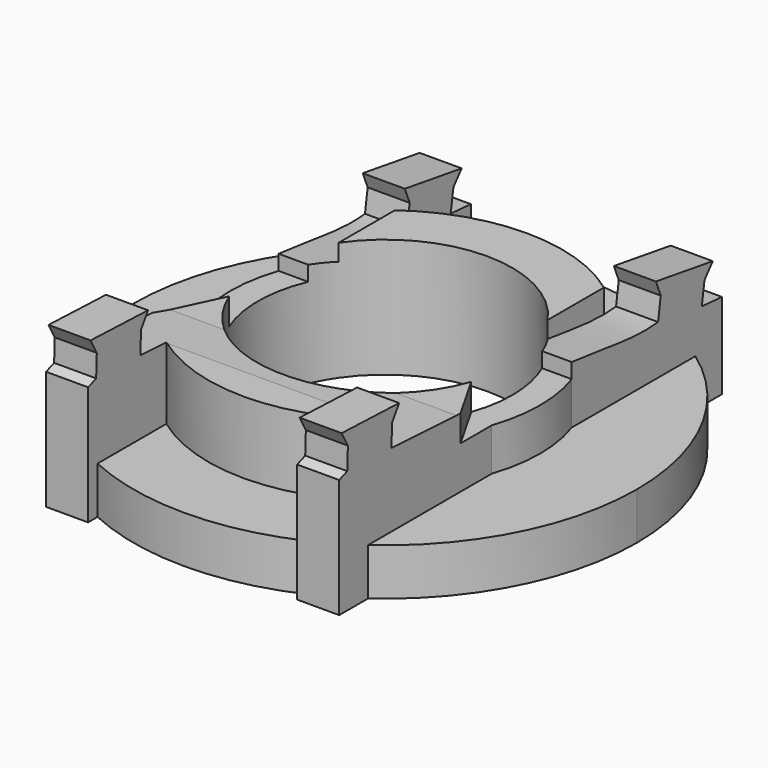
from build123d import *
from build123d import SkipClean  # not in build123d's __all__

# Parameters (mm, degrees)
F2_DEPTH = 8.5
F3_DEPTH = 29
F4_DEPTH = 16.2
F5_DEPTH = 21.5
F6_W     = 8.4938306999
F6_H     = 8
F7_DEPTH = 53
F8_DEPTH = 7.6
F9_START = -45.4
F9_DEPTH = 9.2


with BuildPart() as f2:
    # F0 (on Top) → F2 (new body)
    with BuildSketch(Plane.XY):
        with BuildLine():
            ThreePointArc((-26.5, -9.04157066), (-28, 0), (-26.5, 9.04157066))
            Line((-26.5, 9.04157066), (-26.5, 36.9864840178))
            ThreePointArc((-26.5, 36.9864840178), (-45.5, 0), (-26.5, -36.9864840178))
            Line((-26.5, -36.9864840178), (-26.5, -19.535109446))
            Line((-26.5, -19.535109446), (-26.5, -9.04157066))
        make_face()
        with BuildLine():
            Line((18.9, -41.3888873975), (18.9, -25.822277204))
            ThreePointArc((18.9, -25.822277204), (0, -32), (-18.9, -25.822277204))
            Line((-18.9, -25.822277204), (-18.9, -41.3888873975))
            ThreePointArc((-18.9, -41.3888873975), (0, -45.5), (18.9, -41.3888873975))
        make_face()
        with BuildLine():
            Line((26.5, 36.9864840178), (26.5, 9.04157066))
            ThreePointArc((26.5, 9.04157066), (28, 0), (26.5, -9.04157066))
            Line((26.5, -9.04157066), (26.5, -16.0938306999))
            Line((26.5, -16.0938306999), (26.5, -36.9864840178))
            ThreePointArc((26.5, -36.9864840178), (40.4722126897, -20.7906228863), (45.5, 0))
            ThreePointArc((45.5, 0), (40.4722126897, 20.7906228863), (26.5, 36.9864840178))
        make_face()
        with BuildLine():
            ThreePointArc((-18.9, 25.822277204), (0, 32), (18.9, 25.822277204))
            Line((18.9, 25.822277204), (18.9, 41.3888873975))
            ThreePointArc((18.9, 41.3888873975), (0, 45.5), (-18.9, 41.3888873975))
            Line((-18.9, 41.3888873975), (-18.9, 25.822277204))
        make_face()
        with BuildLine():
            Line((-18.9, -25.822277204), (-18.9, -13.1068684284))
            ThreePointArc((-18.9, -13.1068684284), (-20.2445385279, -10.915981852), (-21.3362014212, -8.588743151))
            Line((-21.3362014212, -8.588743151), (-26.5, -19.535109446))
            Line((-26.5, -19.535109446), (-26.5, -36.9864840178))
            ThreePointArc((-26.5, -36.9864840178), (-22.806474714, -39.3714961758), (-18.9, -41.3888873975))
            Line((-18.9, -41.3888873975), (-18.9, -25.822277204))
        make_face()
        with BuildLine():
            Line((18.9, -25.822277204), (18.9, -13.1068684284))
            ThreePointArc((18.9, -13.1068684284), (0, -23), (-18.9, -13.1068684284))
            Line((-18.9, -13.1068684284), (-18.9, -25.822277204))
            ThreePointArc((-18.9, -25.822277204), (0, -32), (18.9, -25.822277204))
        make_face()
        with BuildLine():
            Line((26.5, -16.0938306999), (21.6892735119, -7.6534576843))
            ThreePointArc((21.6892735119, -7.6534576843), (20.4769920458, -10.4734329022), (18.9, -13.1068684284))
            Line((18.9, -13.1068684284), (18.9, -25.822277204))
            Line((18.9, -25.822277204), (18.9, -41.3888873975))
            ThreePointArc((18.9, -41.3888873975), (22.806474714, -39.3714961758), (26.5, -36.9864840178))
            Line((26.5, -36.9864840178), (26.5, -16.0938306999))
        make_face()
        with BuildLine():
            ThreePointArc((21.1482859826, 9.04157066), (22.5323165431, 4.614619291), (23, 0))
            ThreePointArc((23, 0), (22.6699502731, -3.8824418364), (21.6892735119, -7.6534576843))
            Line((21.6892735119, -7.6534576843), (26.5, -16.0938306999))
            Line((26.5, -16.0938306999), (26.5, -9.04157066))
            ThreePointArc((26.5, -9.04157066), (28, 0), (26.5, 9.04157066))
            Line((26.5, 9.04157066), (21.1482859826, 9.04157066))
        make_face()
        with BuildLine():
            ThreePointArc((18.9, 13.1068684284), (20.127045586, 11.1311291421), (21.1482859826, 9.04157066))
            Line((21.1482859826, 9.04157066), (26.5, 9.04157066))
            Line((26.5, 9.04157066), (26.5, 36.9864840178))
            ThreePointArc((26.5, 36.9864840178), (22.806474714, 39.3714961758), (18.9, 41.3888873975))
            Line((18.9, 41.3888873975), (18.9, 25.822277204))
            Line((18.9, 25.822277204), (18.9, 13.1068684284))
        make_face()
        with BuildLine():
            ThreePointArc((-18.9, 13.1068684284), (0, 23), (18.9, 13.1068684284))
            Line((18.9, 13.1068684284), (18.9, 25.822277204))
            ThreePointArc((18.9, 25.822277204), (0, 32), (-18.9, 25.822277204))
            Line((-18.9, 25.822277204), (-18.9, 13.1068684284))
        make_face()
        with BuildLine():
            ThreePointArc((-21.1482859826, 9.04157066), (-20.127045586, 11.1311291421), (-18.9, 13.1068684284))
            Line((-18.9, 13.1068684284), (-18.9, 25.822277204))
            Line((-18.9, 25.822277204), (-18.9, 41.3888873975))
            ThreePointArc((-18.9, 41.3888873975), (-22.806474714, 39.3714961758), (-26.5, 36.9864840178))
            Line((-26.5, 36.9864840178), (-26.5, 9.04157066))
            Line((-26.5, 9.04157066), (-21.1482859826, 9.04157066))
        make_face()
        with BuildLine():
            ThreePointArc((-21.3362014212, -8.588743151), (-22.9986936316, 0.245135149), (-21.1482859826, 9.04157066))
            Line((-21.1482859826, 9.04157066), (-26.5, 9.04157066))
            ThreePointArc((-26.5, 9.04157066), (-28, 0), (-26.5, -9.04157066))
            Line((-26.5, -9.04157066), (-26.5, -19.535109446))
            Line((-26.5, -19.535109446), (-21.3362014212, -8.588743151))
        make_face()
        with BuildLine():
            ThreePointArc((-26.5, 36.9864840178), (-22.806474714, 39.3714961758), (-18.9, 41.3888873975))
            Line((-18.9, 41.3888873975), (-18.9, 42.9887993038))
            Line((-18.9, 42.9887993038), (-26.5, 42.9887993038))
            Line((-26.5, 42.9887993038), (-26.5, 36.9864840178))
        make_face()
        with BuildLine():
            ThreePointArc((18.9, 41.3888873975), (22.806474714, 39.3714961758), (26.5, 36.9864840178))
            Line((26.5, 36.9864840178), (26.5, 42.9887993038))
            Line((26.5, 42.9887993038), (18.9, 42.9887993038))
            Line((18.9, 42.9887993038), (18.9, 41.3888873975))
        make_face()
        with BuildLine():
            Line((26.5, -43.5112006962), (26.5, -36.9864840178))
            ThreePointArc((26.5, -36.9864840178), (22.806474714, -39.3714961758), (18.9, -41.3888873975))
            Line((18.9, -41.3888873975), (18.9, -43.5112006962))
            Line((18.9, -43.5112006962), (26.5, -43.5112006962))
        make_face()
        with BuildLine():
            Line((-18.9, -43.5112006962), (-18.9, -41.3888873975))
            ThreePointArc((-18.9, -41.3888873975), (-22.806474714, -39.3714961758), (-26.5, -36.9864840178))
            Line((-26.5, -36.9864840178), (-26.5, -43.5112006962))
            Line((-26.5, -43.5112006962), (-18.9, -43.5112006962))
        make_face()
    extrude(amount=F2_DEPTH)

    # F0 (on Top) → F3 (join)
    with BuildSketch(Plane.XY):
        with BuildLine():
            Line((-18.9, -25.822277204), (-18.9, -13.1068684284))
            ThreePointArc((-18.9, -13.1068684284), (-20.2445385279, -10.915981852), (-21.3362014212, -8.588743151))
            Line((-21.3362014212, -8.588743151), (-26.5, -19.535109446))
            Line((-26.5, -19.535109446), (-26.5, -36.9864840178))
            ThreePointArc((-26.5, -36.9864840178), (-22.806474714, -39.3714961758), (-18.9, -41.3888873975))
            Line((-18.9, -41.3888873975), (-18.9, -25.822277204))
        make_face()
        with BuildLine():
            ThreePointArc((-21.1482859826, 9.04157066), (-20.127045586, 11.1311291421), (-18.9, 13.1068684284))
            Line((-18.9, 13.1068684284), (-18.9, 25.822277204))
            Line((-18.9, 25.822277204), (-18.9, 41.3888873975))
            ThreePointArc((-18.9, 41.3888873975), (-22.806474714, 39.3714961758), (-26.5, 36.9864840178))
            Line((-26.5, 36.9864840178), (-26.5, 9.04157066))
            Line((-26.5, 9.04157066), (-21.1482859826, 9.04157066))
        make_face()
        with BuildLine():
            ThreePointArc((18.9, 13.1068684284), (20.127045586, 11.1311291421), (21.1482859826, 9.04157066))
            Line((21.1482859826, 9.04157066), (26.5, 9.04157066))
            Line((26.5, 9.04157066), (26.5, 36.9864840178))
            ThreePointArc((26.5, 36.9864840178), (22.806474714, 39.3714961758), (18.9, 41.3888873975))
            Line((18.9, 41.3888873975), (18.9, 25.822277204))
            Line((18.9, 25.822277204), (18.9, 13.1068684284))
        make_face()
        with BuildLine():
            Line((26.5, -16.0938306999), (21.6892735119, -7.6534576843))
            ThreePointArc((21.6892735119, -7.6534576843), (20.4769920458, -10.4734329022), (18.9, -13.1068684284))
            Line((18.9, -13.1068684284), (18.9, -25.822277204))
            Line((18.9, -25.822277204), (18.9, -41.3888873975))
            ThreePointArc((18.9, -41.3888873975), (22.806474714, -39.3714961758), (26.5, -36.9864840178))
            Line((26.5, -36.9864840178), (26.5, -16.0938306999))
        make_face()
        with BuildLine():
            Line((-18.9, -43.5112006962), (-18.9, -41.3888873975))
            ThreePointArc((-18.9, -41.3888873975), (-22.806474714, -39.3714961758), (-26.5, -36.9864840178))
            Line((-26.5, -36.9864840178), (-26.5, -43.5112006962))
            Line((-26.5, -43.5112006962), (-18.9, -43.5112006962))
        make_face()
        with BuildLine():
            Line((26.5, -43.5112006962), (26.5, -36.9864840178))
            ThreePointArc((26.5, -36.9864840178), (22.806474714, -39.3714961758), (18.9, -41.3888873975))
            Line((18.9, -41.3888873975), (18.9, -43.5112006962))
            Line((18.9, -43.5112006962), (26.5, -43.5112006962))
        make_face()
        with BuildLine():
            ThreePointArc((18.9, 41.3888873975), (22.806474714, 39.3714961758), (26.5, 36.9864840178))
            Line((26.5, 36.9864840178), (26.5, 42.9887993038))
            Line((26.5, 42.9887993038), (18.9, 42.9887993038))
            Line((18.9, 42.9887993038), (18.9, 41.3888873975))
        make_face()
        with BuildLine():
            ThreePointArc((-26.5, 36.9864840178), (-22.806474714, 39.3714961758), (-18.9, 41.3888873975))
            Line((-18.9, 41.3888873975), (-18.9, 42.9887993038))
            Line((-18.9, 42.9887993038), (-26.5, 42.9887993038))
            Line((-26.5, 42.9887993038), (-26.5, 36.9864840178))
        make_face()
    with SkipClean():  # cleaning this boolean's faces spoils the solid; the shape is the same uncleaned
        extrude(amount=F3_DEPTH)

    # F0 (on Top) → F4 (join)
    with BuildSketch(Plane.XY):
        with BuildLine():
            ThreePointArc((-21.3362014212, -8.588743151), (-22.9986936316, 0.245135149), (-21.1482859826, 9.04157066))
            Line((-21.1482859826, 9.04157066), (-26.5, 9.04157066))
            ThreePointArc((-26.5, 9.04157066), (-28, 0), (-26.5, -9.04157066))
            Line((-26.5, -9.04157066), (-26.5, -19.535109446))
            Line((-26.5, -19.535109446), (-21.3362014212, -8.588743151))
        make_face()
        with BuildLine():
            ThreePointArc((21.1482859826, 9.04157066), (22.5323165431, 4.614619291), (23, 0))
            ThreePointArc((23, 0), (22.6699502731, -3.8824418364), (21.6892735119, -7.6534576843))
            Line((21.6892735119, -7.6534576843), (26.5, -16.0938306999))
            Line((26.5, -16.0938306999), (26.5, -9.04157066))
            ThreePointArc((26.5, -9.04157066), (28, 0), (26.5, 9.04157066))
            Line((26.5, 9.04157066), (21.1482859826, 9.04157066))
        make_face()
    extrude(amount=F4_DEPTH)

    # F0 (on Top) → F5 (join)
    with BuildSketch(Plane.XY):
        with BuildLine():
            ThreePointArc((-18.9, 13.1068684284), (0, 23), (18.9, 13.1068684284))
            Line((18.9, 13.1068684284), (18.9, 25.822277204))
            ThreePointArc((18.9, 25.822277204), (0, 32), (-18.9, 25.822277204))
            Line((-18.9, 25.822277204), (-18.9, 13.1068684284))
        make_face()
        with BuildLine():
            Line((18.9, -25.822277204), (18.9, -13.1068684284))
            ThreePointArc((18.9, -13.1068684284), (0, -23), (-18.9, -13.1068684284))
            Line((-18.9, -13.1068684284), (-18.9, -25.822277204))
            ThreePointArc((-18.9, -25.822277204), (0, -32), (18.9, -25.822277204))
        make_face()
    extrude(amount=F5_DEPTH)

    # F6 (on face) → F7 (cut)
    with BuildSketch(Plane.YZ.offset(26.5)):
        Polygon((-31.7034486039, 21.8143278533), (-17, 21), (-16.0938306999, 21), (-16.0938306999, 29), (-43.5112006962, 29), (-43.5112006962, 21.5072025748), (-41.6965513961, 22.1856721467), (-41.5480136787, 26.1829132636), (-42.9539764288, 28.7413737907), (-29.9629427989, 28.2586262093), (-31.5549108865, 25.8115689702), align=None)
        with Locations((-11.8469153499, 25)):
            Rectangle(F6_W, F6_H)
    extrude(amount=-F7_DEPTH, mode=Mode.SUBTRACT)

    # F6 (on face) → F8 (cut, through all)
    with BuildSketch(Plane.YZ.offset(26.5)):
        with BuildLine():
            Line((38.4415975598, 15.8380199759), (43, 15.5))
            Line((43, 15.5), (43, 29))
            Line((43, 29), (8.2, 29))
            Line((8.2, 29), (8.2, 19))
            add(Edge.make_bspline(
                [(28.5584024402, 17.3619800241), (22.9, 16.6746068906), (15.6, 18.3999594301), (8.2, 19)],
                knots=[0, 0, 0, 0, 20.4241929916, 20.4241929916, 20.4241929916, 20.4241929916], degree=3))
            Line((28.5584024402, 17.3619800241), (29.1679864595, 21.3152580719))
            Line((29.1679864595, 21.3152580719), (28.0664972036, 24.014650859))
            Line((28.0664972036, 24.014650859), (40.914650859, 22.0335027964))
            Line((40.914650859, 22.0335027964), (39.051181579, 19.7912980238))
            Line((39.051181579, 19.7912980238), (38.4415975598, 15.8380199759))
        make_face()
    extrude(amount=-F8_DEPTH, mode=Mode.SUBTRACT)

    # F6 (on face) → F9 (cut)
    with BuildSketch(Plane.YZ.offset(26.5).offset(F9_START)):
        with BuildLine():
            Line((38.4415975598, 15.8380199759), (43, 15.5))
            Line((43, 15.5), (43, 29))
            Line((43, 29), (8.2, 29))
            Line((8.2, 29), (8.2, 19))
            add(Edge.make_bspline(
                [(28.5584024402, 17.3619800241), (22.9, 16.6746068906), (15.6, 18.3999594301), (8.2, 19)],
                knots=[0, 0, 0, 0, 20.4241929916, 20.4241929916, 20.4241929916, 20.4241929916], degree=3))
            Line((28.5584024402, 17.3619800241), (29.1679864595, 21.3152580719))
            Line((29.1679864595, 21.3152580719), (28.0664972036, 24.014650859))
            Line((28.0664972036, 24.014650859), (40.914650859, 22.0335027964))
            Line((40.914650859, 22.0335027964), (39.051181579, 19.7912980238))
            Line((39.051181579, 19.7912980238), (38.4415975598, 15.8380199759))
        make_face()
    extrude(amount=-F9_DEPTH, mode=Mode.SUBTRACT)


solid = f2.part
